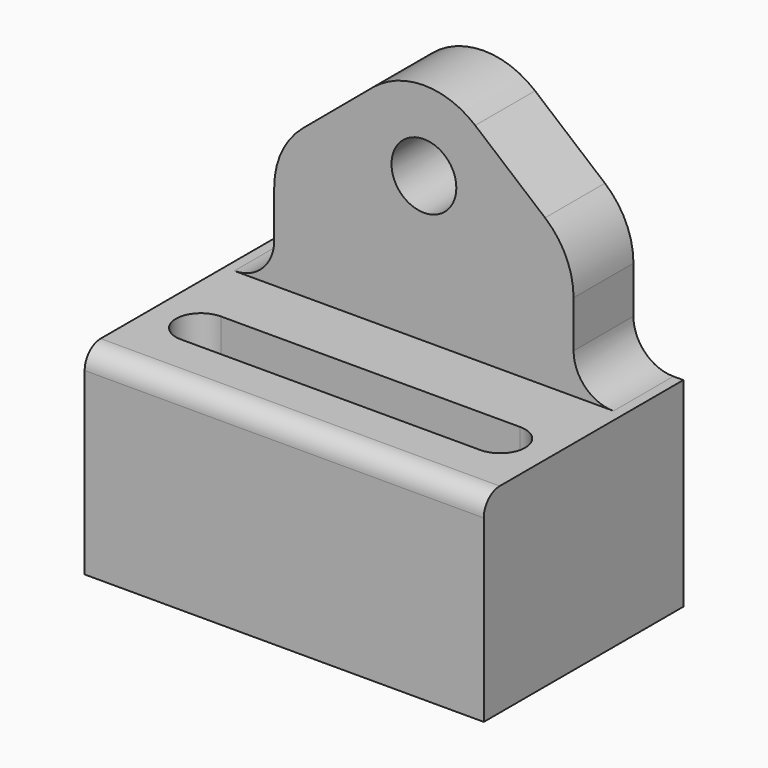
from build123d import *

# Parameters (mm, degrees)
F0_W      = 101.6
F0_H      = 63.5
F1_DEPTH  = 50.8
F2_R      = 5.08
F4_DEPTH  = 12.7
F5_W      = 101.6
F5_H      = 19.05
F6_DEPTH  = 63.5
F8_DEPTH  = 25.4
F9_R      = 20.32
F10_R     = 10.16
F11_R     = 8.255
F12_DEPTH = 25.4


with BuildPart() as f1:
    # F0 (on Top) → F1 (new body)
    with BuildSketch(Plane.XY):
        with Locations((0, -6.35)):
            Rectangle(F0_W, F0_H)
    extrude(amount=F1_DEPTH)

    # F2
    f2_edges = [f1.edges().sort_by_distance(p)[0] for p in [
        (0, -38.1, 50.8),
    ]]
    fillet(f2_edges, radius=F2_R)

    # F3 (on face) → F4 (cut)
    with BuildSketch(Plane.XY.offset(50.8)):
        with BuildLine():
            Line((38.1, -10.6305400074), (-38.1, -10.6305400074))
            ThreePointArc((-38.1, -10.6305400074), (-44.45, -16.9805400074), (-38.1, -23.3305400074))
            Line((-38.1, -23.3305400074), (38.1, -23.3305400074))
            ThreePointArc((38.1, -23.3305400074), (44.45, -16.9805400074), (38.1, -10.6305400074))
        make_face()
    extrude(amount=-F4_DEPTH, mode=Mode.SUBTRACT)

    # F5 (on face) → F6 (join)
    with BuildSketch(Plane.XY.offset(50.8)):
        with Locations((0, 15.875)):
            Rectangle(F5_W, F5_H)
    extrude(amount=F6_DEPTH)

    # F7 (on face) → F8 (cut)
    with BuildSketch(Plane.XZ.offset(-6.35)):
        Polygon((-50.8, 50.8), (-38.1, 50.8), (-38.1, 82.3303040521), (0, 114.3), (-50.8, 114.3), align=None)
        Polygon((38.1, 50.8), (50.8, 50.8), (50.8, 114.3), (0, 114.3), (38.1, 82.3303040521), align=None)
    extrude(amount=-F8_DEPTH, mode=Mode.SUBTRACT)

    # F9
    f9_edges = [f1.edges().sort_by_distance(p)[0] for p in [
        (38.1, 15.875, 82.330304),
        (-38.1, 15.875, 82.330304),
        (0, 15.875, 114.3),
    ]]
    fillet(f9_edges, radius=F9_R)

    # F10
    f10_edges = [f1.edges().sort_by_distance(p)[0] for p in [
        (38.1, 15.875, 50.8),
        (-38.1, 15.875, 50.8),
    ]]
    fillet(f10_edges, radius=F10_R)

    # F11 (on face) → F12 (cut)
    with BuildSketch(Plane.XZ.offset(-6.35)):
        with Locations((0, 87.7741238808)):
            Circle(F11_R)
    extrude(amount=-F12_DEPTH, mode=Mode.SUBTRACT)


solid = f1.part
